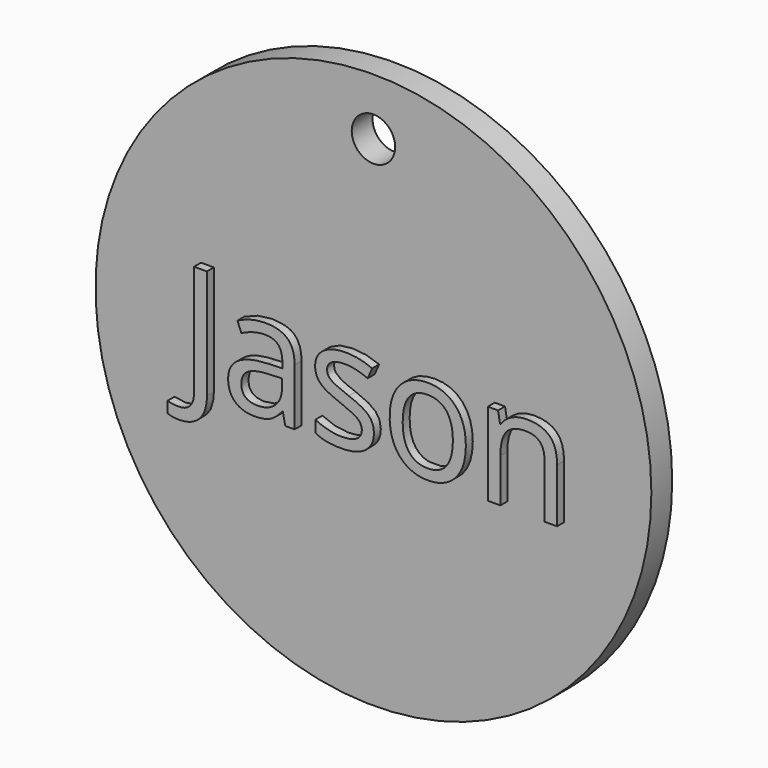
from build123d import *

# Parameters (mm, degrees)
F0_TEXT_SIZE = 22.6392976082
F1_DEPTH     = 5.08
F2_R         = 40.64
F3_DEPTH     = 3.81
F5_D         = 6.35


# Not quite as in the source:
# - Text() gives the source's letters only with a copy of the font that has no kerning and outlines rounded to 1/6400 em; it was checked with that copy


with BuildPart() as f1:
    # F0 (on Front) → F1 (new body)
    with BuildSketch(Plane.XZ):
        with Locations((-27.3127155704, -7.9731067419)):
            Text('Jason', F0_TEXT_SIZE, font='Open Sans', text_align=(TextAlign.LEFT, TextAlign.BOTTOM))
    extrude(amount=F1_DEPTH)


with BuildPart() as f3:
    # F2 (on Front) → F3 (new body)
    with BuildSketch(Plane.XZ):
        Circle(F2_R)
    extrude(amount=F3_DEPTH)

    # F5 (through all)
    with Locations(Plane(origin=(0, 0, 0), x_dir=(1, 0, 0), z_dir=(0, 1, 0))):
        with Locations((0, -32.3017053306)):
            Hole(F5_D / 2)


solid = Compound([f1.part, f3.part])
